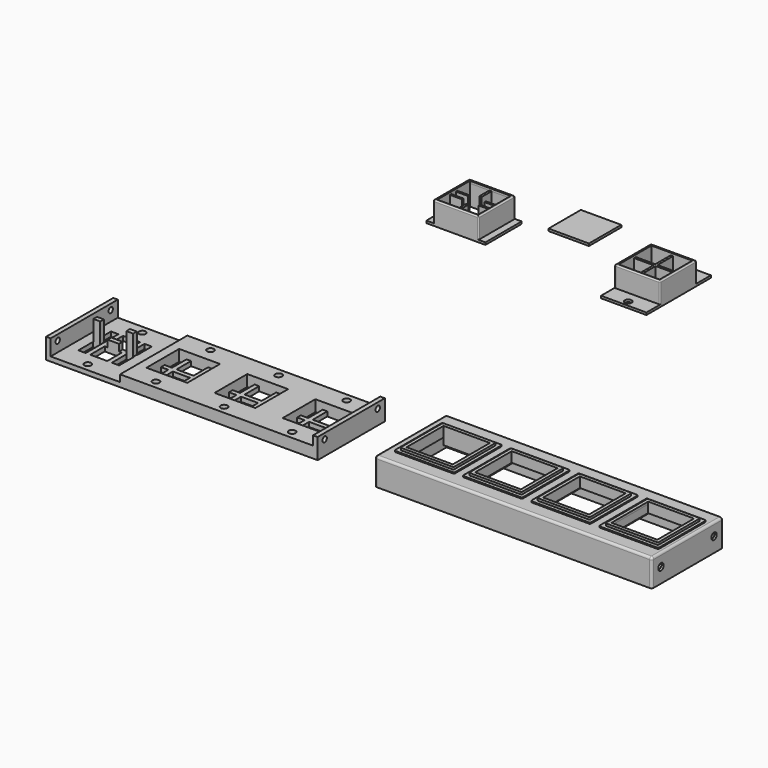
from build123d import *

# Parameters (mm, degrees)
F0_W          = 20
F0_H          = 20
F1_DEPTH      = 10
F2_T          = -1
F4_DEPTH      = 9
F5_W          = 20
F5_H          = 8
F5_R          = 1.5
F6_DEPTH      = 1
F7_W          = 20
F7_H          = 20
F8_DEPTH      = 10
F9_W          = 3
F9_H          = 20
F9_W_2        = 20
F10_DEPTH     = 0.95
F11_T         = 1
F11_T3_DEPTH  = 22
F12_W         = 8.5
F12_H         = 0.8
F13_DEPTH     = 9
F15_DEPTH     = 9
F16_W         = 117
F16_H         = 37
F16_R         = 1.5
F17_DEPTH     = 1
F18_W         = 122
F18_H         = 39.2
F18_W_2       = 20.4
F18_H_2       = 20.4
F18_W_3       = 20.2
F18_H_3       = 20.2
F19_DEPTH     = 11
F20_W         = 120
F20_H         = 37.2
F21_DEPTH     = 8
F22_W         = 4
F22_H         = 18
F23_DEPTH     = 3
F25_W         = 3
F25_H         = 2
F26_DEPTH     = 9
F27_W         = 5
F27_H         = 2
F28_DEPTH     = 3
F29_R         = 1
F30_R         = 0.5
F30_2_R       = 0.5
F24_R         = 1.5
F31_DEPTH     = 3
F32_DEPTH     = 2
F33_W         = 2
F33_H         = 37
F34_DEPTH     = 7
F35_W         = 20.4
F35_H         = 8.4
F36_DEPTH     = 3
F37_R         = 1.5
F38_DEPTH     = 3
F40_R         = 1.5
F41_DEPTH     = 2
F42_W         = 3
F42_H         = 37.2
F43_DEPTH     = 1
F44_DEPTH     = 1
F45_W         = 2
F45_H         = 37
F46_DEPTH     = 4
F39_R         = 1.2
F47_DEPTH     = 269.2358512024
F48_DEPTH     = 3
F49_DEPTH     = 5
F32_FACE2_W   = 119
F32_FACE2_H   = 37
F32_FACE2_R   = 1.5
F32_FACE2_W_2 = 3.25
F32_FACE2_H_2 = 8
F32_FACE2_W_3 = 7.5
F50_DEPTH     = 1
F51_DEPTH     = 1
F52_DEPTH     = 2
F53_DEPTH     = 0.05
F54_W         = 20.4
F54_H         = 3
F54_W_2       = 20.2
F54_H_2       = 3.1
F55_DEPTH     = 0.5
F56_W         = 20.4
F56_H         = 1.5
F56_W_2       = 20.2
F57_DEPTH     = 1
F58_R         = 0.5
F59_W         = 18
F59_H         = 17.9999990673
F60_DEPTH     = 1
F61_W         = 17.8
F61_H         = 17.8
F62_DEPTH     = 1
F63_W         = 18
F63_H         = 18
F64_DEPTH     = 1


# Not quite as in the source:
# - a shell that OpenCascade refuses in one call is made with other operations: the cavity is built on its own and cut out


with BuildPart() as f1:
    # F0 (on Top) → F1 (new body)
    with BuildSketch(Plane.XY):
        Rectangle(F0_W, F0_H)
    extrude(amount=F1_DEPTH)

    # F2
    f2_openings = [f1.faces().sort_by_distance(p)[0] for p in [
        (0, 0, 0),
    ]]
    offset(amount=F2_T, openings=f2_openings)

    # F3 (on Top) → F4 (join)
    with BuildSketch(Plane.XY):
        Polygon((-0.5, -9), (0.5, -9), (0.5, -0.5), (9, -0.5), (9, 0.5), (0.5, 0.5), (0.5, 9), (-0.5, 9), (-0.5, 0.5), (-9, 0.5), (-9, -0.5), (-0.5, -0.5), align=None)
    extrude(amount=F4_DEPTH)

    # F5 (on Top) → F6 (join)
    with BuildSketch(Plane.XY):
        with Locations((0, -13.5)):
            Rectangle(F5_W, F5_H)
        with Locations((0, -15)):
            Circle(F5_R, mode=Mode.SUBTRACT)
        with Locations((0, 14)):
            Rectangle(F5_W, F5_H)
        with Locations((0, 15)):
            Circle(F5_R, mode=Mode.SUBTRACT)
    extrude(amount=F6_DEPTH)

    # F30
    f30_edges = [f1.edges().sort_by_distance(p)[0] for p in [
        (-10, -10, 5.5),
        (0, -10, 10),
        (10, -10, 5.5),
        (-10, 0, 10),
        (-10, 10, 5.5),
        (0, 10, 10),
        (10, 10, 5.5),
        (10, 0, 10),
    ]]
    fillet(f30_edges, radius=F30_R)

    # F63 (on face) → F64 (cut)
    with BuildSketch(Plane.XY.offset(10)):
        Rectangle(F63_W, F63_H)
    extrude(amount=-F64_DEPTH, mode=Mode.SUBTRACT)


with BuildPart() as f8:
    # F7 (on Top) → F8 (new body)
    with BuildSketch(Plane.XY):
        with Locations((-78.8846665621, -1.3073290847)):
            Rectangle(F7_W, F7_H)
    extrude(amount=F8_DEPTH)

    # F9 (on face) → F10 (join)
    with BuildSketch(Plane(origin=(0, 0, 0), x_dir=(1, 0, 0), z_dir=(0, 0, -1))):
        with Locations((-90.3846665621, 1.3073290847)):
            Rectangle(F9_W, F9_H)
        with Locations((-78.8846665621, 1.3073290847)):
            Rectangle(F9_W_2, F9_H)
        with Locations((-67.3846665621, 1.3073290847)):
            Rectangle(F9_W, F9_H)
    extrude(amount=-F10_DEPTH)

    # F11: shell of thickness 1, made by hand


with BuildPart() as f11_core1:
    # F11_t2: copy of F8
    add(f8.part)

    # the walls: a layer under each face that stays
    f11_faces = [f11_core1.faces().sort_by_distance(p)[0] for p in [
        (-78.8846665621, 8.6926709153, 5),
        (-91.8846665621, -1.3073290847, 0.475),
        (-78.8846665621, -11.3073290847, 5),
        (-90.3846665621, -1.3073290847, 0.95),
        (-88.8846665621, -1.3073290847, 5.475),
        (-78.8846665621, -1.3073290847, 10),
        (-68.8846665621, -1.3073290847, 5.475),
        (-67.3846665621, -1.3073290847, 0.95),
        (-65.8846665621, -1.3073290847, 0.475),
    ]]
    thicken(f11_faces, amount=-F11_T, mode=Mode.SUBTRACT)

    # F11_s4 → F11_t3 (cut)
    with BuildSketch(Plane.XZ.offset(-9.6926709153)):
        Polygon((-88.8946665621, 0.96), (-88.8846665621, -0.05), (-87.8846665621, -0.05), (-87.8846665621, 0.95), align=None)
        Polygon((-68.8746665621, 0.96), (-69.8846665621, 0.95), (-69.8846665621, -0.05), (-68.8846665621, -0.05), align=None)
    extrude(amount=F11_T3_DEPTH, mode=Mode.SUBTRACT)


with BuildPart() as f8_1:
    add(f8.part)

    # what is left inside the walls is the cavity
    f11_cavity = [f11_core1.part.solids().sort_by_distance(p)[0] for p in [
        (-78.884667, -4.307329, 0.01),
    ]]
    add(f11_cavity, mode=Mode.SUBTRACT)

    # F12 (on Top) → F13 (join)
    with BuildSketch(Plane.XY):
        Polygon((-78.3846665621, 7.6926709153), (-79.3846665621, 7.6926709153), (-79.3846665621, 0.6926709153), (-79.3846665621, -0.1073290847), (-79.3846665621, -2.5073290847), (-79.3846665621, -3.3073290847), (-79.3846665621, -10.3073290847), (-78.3846665621, -10.3073290847), (-78.3846665621, -3.3073290847), (-78.3846665621, -2.5073290847), (-78.3846665621, -0.1073290847), (-78.3846665621, 0.6926709153), align=None)
        with Locations((-83.6346665621, -2.9073290847)):
            Rectangle(F12_W, F12_H)
        with Locations((-83.6346665621, 0.2926709153)):
            Rectangle(F12_W, F12_H)
        with Locations((-74.1346665621, 0.2926709153)):
            Rectangle(F12_W, F12_H)
        with Locations((-74.1346665621, -2.9073290847)):
            Rectangle(F12_W, F12_H)
    extrude(amount=F13_DEPTH)

    # F14 (on face) → F15 (cut)
    with BuildSketch(Plane(origin=(0, 0, 0), x_dir=(1, 0, 0), z_dir=(0, 0, -1))):
        Polygon((-79.3846665621, -2.2926709153), (-78.3846665621, -2.2926709153), (-78.3846665621, -0.6926709153), (-75.2846665621, -0.6926709153), (-75.2846665621, 0.1073290847), (-78.3846665621, 0.1073290847), (-78.3846665621, 2.5073290847), (-75.2846665621, 2.5073290847), (-75.2846665621, 3.3073290847), (-78.3846665621, 3.3073290847), (-78.3846665621, 4.9073290847), (-79.3846665621, 4.9073290847), (-79.3846665621, 3.3073290847), (-82.4846665621, 3.3073290847), (-82.4846665621, 2.5073290847), (-79.3846665621, 2.5073290847), (-79.3846665621, 0.1073290847), (-82.4846665621, 0.1073290847), (-82.4846665621, -0.6926709153), (-79.3846665621, -0.6926709153), align=None)
    extrude(amount=-F15_DEPTH, mode=Mode.SUBTRACT)

    # F30#2
    f30_2_edges = [f8_1.edges().sort_by_distance(p)[0] for p in [
        (-68.884667, -11.307329, 5.475),
        (-78.884667, -11.307329, 10),
        (-68.884667, -1.307329, 10),
        (-68.884667, 8.692671, 5.475),
        (-78.884667, 8.692671, 10),
        (-88.884667, 8.692671, 5.475),
        (-88.884667, -1.307329, 10),
        (-88.884667, -11.307329, 5.475),
    ]]
    fillet(f30_2_edges, radius=F30_2_R)

    # F53 (add): faces of the model
    f53_faces = [f8_1.faces().sort_by_distance(p)[0] for p in [
        (-90.3817894545, -1.3073290847, 0.95),
        (-67.3875436696, -1.3073290847, 0.95),
    ]]
    extrude(f53_faces, amount=F53_DEPTH)

    # F59 (on face) → F60 (cut)
    with BuildSketch(Plane.XY.offset(10)):
        with Locations((-78.8846665621, -1.3073295511)):
            Rectangle(F59_W, F59_H)
    extrude(amount=-F60_DEPTH, mode=Mode.SUBTRACT)


with BuildPart() as f17:
    # F16 (on Top) → F17 (new body)
    with BuildSketch(Plane.XY):
        with Locations((-71.0754835367, -152.5580135584)):
            Rectangle(F16_W, F16_H)
        with Locations((-115.9754835367, -167.5580135584)):
            Circle(F16_R, mode=Mode.SUBTRACT)
        with Locations((-85.9754835367, -167.5580135584)):
            Circle(F16_R, mode=Mode.SUBTRACT)
        Polygon((-124.9754835367, -151.5580135584), (-124.9754835367, -143.5580135584), (-121.7254835367, -143.5580135584), (-119.7254835367, -143.5580135584), (-112.2254835367, -143.5580135584), (-110.2254835367, -143.5580135584), (-106.9754835367, -143.5580135584), (-106.9754835367, -151.5580135584), (-106.9754835367, -153.5580135584), (-106.9754835367, -161.5580135584), (-110.2254835367, -161.5580135584), (-112.2254835367, -161.5580135584), (-119.7254835367, -161.5580135584), (-121.7254835367, -161.5580135584), (-124.9754835367, -161.5580135584), (-124.9754835367, -153.5580135584), align=None, mode=Mode.SUBTRACT)
        Polygon((-94.9754835367, -151.5580135584), (-94.9754835367, -143.5580135584), (-91.7254835367, -143.5580135584), (-89.7254835367, -143.5580135584), (-82.2254835367, -143.5580135584), (-80.2254835367, -143.5580135584), (-76.9754835367, -143.5580135584), (-76.9754835367, -151.5580135584), (-76.9754835367, -153.5580135584), (-76.9754835367, -161.5580135584), (-80.2254835367, -161.5580135584), (-82.2254835367, -161.5580135584), (-89.7254835367, -161.5580135584), (-91.7254835367, -161.5580135584), (-94.9754835367, -161.5580135584), (-94.9754835367, -153.5580135584), align=None, mode=Mode.SUBTRACT)
        with Locations((-55.9754835367, -167.5580135584)):
            Circle(F16_R, mode=Mode.SUBTRACT)
        with Locations((-25.9754835367, -167.5580135584)):
            Circle(F16_R, mode=Mode.SUBTRACT)
        Polygon((-64.9754835367, -151.5580135584), (-64.9754835367, -143.5580135584), (-61.7254835367, -143.5580135584), (-59.7254835367, -143.5580135584), (-52.2254835367, -143.5580135584), (-50.2254835367, -143.5580135584), (-46.9754835367, -143.5580135584), (-46.9754835367, -151.5580135584), (-46.9754835367, -153.5580135584), (-46.9754835367, -161.5580135584), (-47.9754835367, -161.5580135584), (-50.2254835367, -161.5580135584), (-52.2254835367, -161.5580135584), (-59.7254835367, -161.5580135584), (-61.7254835367, -161.5580135584), (-64.9754835367, -161.5580135584), (-64.9754835367, -153.5580135584), align=None, mode=Mode.SUBTRACT)
        Polygon((-34.9754835367, -151.5580135584), (-34.9754835367, -143.5580135584), (-31.7254835367, -143.5580135584), (-29.7254835367, -143.5580135584), (-22.2254835367, -143.5580135584), (-20.2254835367, -143.5580135584), (-16.9754835367, -143.5580135584), (-16.9754835367, -151.5580135584), (-16.9754835367, -153.5580135584), (-16.9754835367, -161.5580135584), (-17.9754835367, -161.5580135584), (-20.2254835367, -161.5580135584), (-22.2254835367, -161.5580135584), (-29.7254835367, -161.5580135584), (-31.7254835367, -161.5580135584), (-34.9754835367, -161.5580135584), (-34.9754835367, -153.5580135584), align=None, mode=Mode.SUBTRACT)
        with Locations((-115.9754835367, -137.5580135584)):
            Circle(F16_R, mode=Mode.SUBTRACT)
        with Locations((-85.9754835367, -137.5580135584)):
            Circle(F16_R, mode=Mode.SUBTRACT)
        with Locations((-55.9754835367, -137.5580135584)):
            Circle(F16_R, mode=Mode.SUBTRACT)
        with Locations((-25.9754835367, -137.5580135584)):
            Circle(F16_R, mode=Mode.SUBTRACT)
        Polygon((-119.7254835367, -143.5580135584), (-121.7254835367, -143.5580135584), (-121.7254835367, -151.5580135584), (-124.9754835367, -151.5580135584), (-124.9754835367, -153.5580135584), (-121.7254835367, -153.5580135584), (-121.7254835367, -161.5580135584), (-119.7254835367, -161.5580135584), (-119.7254835367, -153.5580135584), (-112.2254835367, -153.5580135584), (-112.2254835367, -161.5580135584), (-110.2254835367, -161.5580135584), (-110.2254835367, -153.5580135584), (-106.9754835367, -153.5580135584), (-106.9754835367, -151.5580135584), (-110.2254835367, -151.5580135584), (-110.2254835367, -143.5580135584), (-112.2254835367, -143.5580135584), (-112.2254835367, -151.5580135584), (-119.7254835367, -151.5580135584), align=None)
        Polygon((-89.7254835367, -143.5580135584), (-91.7254835367, -143.5580135584), (-91.7254835367, -151.5580135584), (-94.9754835367, -151.5580135584), (-94.9754835367, -153.5580135584), (-91.7254835367, -153.5580135584), (-91.7254835367, -161.5580135584), (-89.7254835367, -161.5580135584), (-89.7254835367, -153.5580135584), (-82.2254835367, -153.5580135584), (-82.2254835367, -161.5580135584), (-80.2254835367, -161.5580135584), (-80.2254835367, -153.5580135584), (-76.9754835367, -153.5580135584), (-76.9754835367, -151.5580135584), (-80.2254835367, -151.5580135584), (-80.2254835367, -143.5580135584), (-82.2254835367, -143.5580135584), (-82.2254835367, -151.5580135584), (-89.7254835367, -151.5580135584), align=None)
        Polygon((-59.7254835367, -143.5580135584), (-61.7254835367, -143.5580135584), (-61.7254835367, -151.5580135584), (-64.9754835367, -151.5580135584), (-64.9754835367, -153.5580135584), (-61.7254835367, -153.5580135584), (-61.7254835367, -161.5580135584), (-59.7254835367, -161.5580135584), (-59.7254835367, -153.5580135584), (-52.2254835367, -153.5580135584), (-52.2254835367, -161.5580135584), (-50.2254835367, -161.5580135584), (-50.2254835367, -153.5580135584), (-46.9754835367, -153.5580135584), (-46.9754835367, -151.5580135584), (-50.2254835367, -151.5580135584), (-50.2254835367, -143.5580135584), (-52.2254835367, -143.5580135584), (-52.2254835367, -151.5580135584), (-59.7254835367, -151.5580135584), align=None)
        Polygon((-29.7254835367, -143.5580135584), (-31.7254835367, -143.5580135584), (-31.7254835367, -151.5580135584), (-34.9754835367, -151.5580135584), (-34.9754835367, -153.5580135584), (-31.7254835367, -153.5580135584), (-31.7254835367, -161.5580135584), (-29.7254835367, -161.5580135584), (-29.7254835367, -153.5580135584), (-22.2254835367, -153.5580135584), (-22.2254835367, -161.5580135584), (-20.2254835367, -161.5580135584), (-20.2254835367, -153.5580135584), (-16.9754835367, -153.5580135584), (-16.9754835367, -151.5580135584), (-20.2254835367, -151.5580135584), (-20.2254835367, -143.5580135584), (-22.2254835367, -143.5580135584), (-22.2254835367, -151.5580135584), (-29.7254835367, -151.5580135584), align=None)
    extrude(amount=F17_DEPTH)

    # F22 (on face) → F23 (join)
    with BuildSketch(Plane.XY.offset(1)):
        with Locations((-96.9754835367, -152.5580135584)):
            Rectangle(F22_W, F22_H)
        with Locations((-74.9754835367, -152.5580135584)):
            Rectangle(F22_W, F22_H)
        with Locations((-66.9754835367, -152.5580135584)):
            Rectangle(F22_W, F22_H)
        with Locations((-44.9754835367, -152.5580135584)):
            Rectangle(F22_W, F22_H)
        with Locations((-36.9754835367, -152.5580135584)):
            Rectangle(F22_W, F22_H)
        with Locations((-14.9754835367, -152.5580135584)):
            Rectangle(F22_W, F22_H)
    extrude(amount=F23_DEPTH)

    # F25 (on face) → F26 (join)
    with BuildSketch(Plane.XY.offset(1)):
        with Locations((-123.2254835367, -152.5580135584)):
            Rectangle(F25_W, F25_H)
        with Locations((-108.7254835367, -152.5580135584)):
            Rectangle(F25_W, F25_H)
    extrude(amount=F26_DEPTH)

    # F27 (on face) → F28 (join)
    with BuildSketch(Plane.XY.offset(1)):
        with Locations((-115.9754835367, -152.5580135584)):
            Rectangle(F27_W, F27_H)
    extrude(amount=F28_DEPTH)

    # F24 (on face) → F31 (join)
    with BuildSketch(Plane.XY.offset(1)):
        Polygon((-98.9754835367, -134.0580135584), (-98.9754835367, -143.5580135584), (-94.9754835367, -143.5580135584), (-91.7254835367, -143.5580135584), (-89.7254835367, -143.5580135584), (-82.2254835367, -143.5580135584), (-80.2254835367, -143.5580135584), (-76.9754835367, -143.5580135584), (-72.9754835367, -143.5580135584), (-72.9754835367, -134.0580135584), align=None)
        with Locations((-85.9754835367, -137.5580135584)):
            Circle(F24_R, mode=Mode.SUBTRACT)
        Polygon((-94.9754835367, -161.5580135584), (-98.9754835367, -161.5580135584), (-98.9754835367, -171.0580135584), (-72.9754835367, -171.0580135584), (-72.9754835367, -161.5580135584), (-76.9754835367, -161.5580135584), (-80.2254835367, -161.5580135584), (-82.2254835367, -161.5580135584), (-89.7254835367, -161.5580135584), (-91.7254835367, -161.5580135584), align=None)
        with Locations((-85.9754835367, -167.5580135584)):
            Circle(F24_R, mode=Mode.SUBTRACT)
        Polygon((-68.9754835367, -161.5580135584), (-68.9754835367, -171.0580135584), (-42.9754835367, -171.0580135584), (-42.9754835367, -161.5580135584), (-46.9754835367, -161.5580135584), (-50.2254835367, -161.5580135584), (-52.2254835367, -161.5580135584), (-59.7254835367, -161.5580135584), (-61.7254835367, -161.5580135584), (-64.9754835367, -161.5580135584), align=None)
        with Locations((-55.9754835367, -167.5580135584)):
            Circle(F24_R, mode=Mode.SUBTRACT)
        Polygon((-42.9754835367, -134.0580135584), (-68.9754835367, -134.0580135584), (-68.9754835367, -143.5580135584), (-64.9754835367, -143.5580135584), (-61.7254835367, -143.5580135584), (-59.7254835367, -143.5580135584), (-52.2254835367, -143.5580135584), (-50.2254835367, -143.5580135584), (-46.9754835367, -143.5580135584), (-42.9754835367, -143.5580135584), align=None)
        with Locations((-55.9754835367, -137.5580135584)):
            Circle(F24_R, mode=Mode.SUBTRACT)
        Polygon((-12.9754835367, -134.0580135584), (-38.9754835367, -134.0580135584), (-38.9754835367, -143.5580135584), (-34.9754835367, -143.5580135584), (-31.7254835367, -143.5580135584), (-29.7254835367, -143.5580135584), (-22.2254835367, -143.5580135584), (-20.2254835367, -143.5580135584), (-16.9754835367, -143.5580135584), (-12.9754835367, -143.5580135584), align=None)
        with Locations((-25.9754835367, -137.5580135584)):
            Circle(F24_R, mode=Mode.SUBTRACT)
        Polygon((-38.9754835367, -161.5580135584), (-38.9754835367, -171.0580135584), (-12.9754835367, -171.0580135584), (-12.9754835367, -161.5580135584), (-16.9754835367, -161.5580135584), (-20.2254835367, -161.5580135584), (-22.2254835367, -161.5580135584), (-29.7254835367, -161.5580135584), (-31.7254835367, -161.5580135584), (-34.9754835367, -161.5580135584), align=None)
        with Locations((-25.9754835367, -167.5580135584)):
            Circle(F24_R, mode=Mode.SUBTRACT)
    extrude(amount=F31_DEPTH)

    # F32 (add): a face of the model
    f32_faces = [f17.faces().sort_by_distance(p)[0] for p in [
        (-129.5754835367, -152.5580135584, 0.5),
    ]]
    extrude(f32_faces, amount=F32_DEPTH)

    # F33 (on face) → F34 (join)
    with BuildSketch(Plane.XY.offset(1)):
        with Locations((-130.5754835367, -152.5580135584)):
            Rectangle(F33_W, F33_H)
    extrude(amount=F34_DEPTH)

    # F44 (add): a face of the model
    f44_faces = [f17.faces().sort_by_distance(p)[0] for p in [
        (-12.9754835367, -152.5580135584, 2.5),
    ]]
    extrude(f44_faces, amount=F44_DEPTH)

    # F45 (on face) → F46 (join)
    with BuildSketch(Plane.XY.offset(4)):
        with Locations((-12.9754835367, -152.5580135584)):
            Rectangle(F45_W, F45_H)
    extrude(amount=F46_DEPTH)

    # F39 (on face) → F47 (cut, through all)
    with BuildSketch(Plane(origin=(-131.5754835367, 0, 0), x_dir=(0, -1, 0), z_dir=(-1, 0, 0))):
        with Locations((137.9580135584, 5.5)):
            Circle(F39_R)
        with Locations((167.1580135584, 5.5)):
            Circle(F39_R)
    extrude(amount=-F47_DEPTH, mode=Mode.SUBTRACT)

    # F49 (add): faces of the model
    f49_faces = [f17.faces().sort_by_distance(p)[0] for p in [
        (-72.9754835367, -152.5580135584, 2.5),
        (-42.9754835367, -152.5580135584, 2.5),
    ]]
    extrude(f49_faces, amount=F49_DEPTH)

    # F16 (on Top) + F32_face2 (on face) → F50 (join)
    with BuildSketch(Plane.XY):
        with Locations((-71.0754835367, -152.5580135584)):
            Rectangle(F16_W, F16_H)
        with Locations((-115.9754835367, -167.5580135584)):
            Circle(F16_R, mode=Mode.SUBTRACT)
        with Locations((-85.9754835367, -167.5580135584)):
            Circle(F16_R, mode=Mode.SUBTRACT)
        Polygon((-124.9754835367, -151.5580135584), (-124.9754835367, -143.5580135584), (-121.7254835367, -143.5580135584), (-119.7254835367, -143.5580135584), (-112.2254835367, -143.5580135584), (-110.2254835367, -143.5580135584), (-106.9754835367, -143.5580135584), (-106.9754835367, -151.5580135584), (-106.9754835367, -153.5580135584), (-106.9754835367, -161.5580135584), (-110.2254835367, -161.5580135584), (-112.2254835367, -161.5580135584), (-119.7254835367, -161.5580135584), (-121.7254835367, -161.5580135584), (-124.9754835367, -161.5580135584), (-124.9754835367, -153.5580135584), align=None, mode=Mode.SUBTRACT)
        Polygon((-94.9754835367, -151.5580135584), (-94.9754835367, -143.5580135584), (-91.7254835367, -143.5580135584), (-89.7254835367, -143.5580135584), (-82.2254835367, -143.5580135584), (-80.2254835367, -143.5580135584), (-76.9754835367, -143.5580135584), (-76.9754835367, -151.5580135584), (-76.9754835367, -153.5580135584), (-76.9754835367, -161.5580135584), (-80.2254835367, -161.5580135584), (-82.2254835367, -161.5580135584), (-89.7254835367, -161.5580135584), (-91.7254835367, -161.5580135584), (-94.9754835367, -161.5580135584), (-94.9754835367, -153.5580135584), align=None, mode=Mode.SUBTRACT)
        with Locations((-55.9754835367, -167.5580135584)):
            Circle(F16_R, mode=Mode.SUBTRACT)
        with Locations((-25.9754835367, -167.5580135584)):
            Circle(F16_R, mode=Mode.SUBTRACT)
        Polygon((-64.9754835367, -151.5580135584), (-64.9754835367, -143.5580135584), (-61.7254835367, -143.5580135584), (-59.7254835367, -143.5580135584), (-52.2254835367, -143.5580135584), (-50.2254835367, -143.5580135584), (-46.9754835367, -143.5580135584), (-46.9754835367, -151.5580135584), (-46.9754835367, -153.5580135584), (-46.9754835367, -161.5580135584), (-47.9754835367, -161.5580135584), (-50.2254835367, -161.5580135584), (-52.2254835367, -161.5580135584), (-59.7254835367, -161.5580135584), (-61.7254835367, -161.5580135584), (-64.9754835367, -161.5580135584), (-64.9754835367, -153.5580135584), align=None, mode=Mode.SUBTRACT)
        Polygon((-34.9754835367, -151.5580135584), (-34.9754835367, -143.5580135584), (-31.7254835367, -143.5580135584), (-29.7254835367, -143.5580135584), (-22.2254835367, -143.5580135584), (-20.2254835367, -143.5580135584), (-16.9754835367, -143.5580135584), (-16.9754835367, -151.5580135584), (-16.9754835367, -153.5580135584), (-16.9754835367, -161.5580135584), (-17.9754835367, -161.5580135584), (-20.2254835367, -161.5580135584), (-22.2254835367, -161.5580135584), (-29.7254835367, -161.5580135584), (-31.7254835367, -161.5580135584), (-34.9754835367, -161.5580135584), (-34.9754835367, -153.5580135584), align=None, mode=Mode.SUBTRACT)
        with Locations((-115.9754835367, -137.5580135584)):
            Circle(F16_R, mode=Mode.SUBTRACT)
        with Locations((-85.9754835367, -137.5580135584)):
            Circle(F16_R, mode=Mode.SUBTRACT)
        with Locations((-55.9754835367, -137.5580135584)):
            Circle(F16_R, mode=Mode.SUBTRACT)
        with Locations((-25.9754835367, -137.5580135584)):
            Circle(F16_R, mode=Mode.SUBTRACT)
    with BuildSketch(Plane(origin=(-72.3791549796, -152.5580135584, 0), x_dir=(1, 0, 0), z_dir=(0, 0, -1))):
        with Locations((0.3036714428, 0)):
            Rectangle(F32_FACE2_W, F32_FACE2_H)
        with Locations((-43.5963285572, 15)):
            Circle(F32_FACE2_R, mode=Mode.SUBTRACT)
        with Locations((-13.5963285572, 15)):
            Circle(F32_FACE2_R, mode=Mode.SUBTRACT)
        with Locations((-36.2213285572, 5)):
            Rectangle(F32_FACE2_W_2, F32_FACE2_H_2, mode=Mode.SUBTRACT)
        with Locations((-43.5963285572, 5)):
            Rectangle(F32_FACE2_W_3, F32_FACE2_H_2, mode=Mode.SUBTRACT)
        with Locations((-50.9713285572, 5)):
            Rectangle(F32_FACE2_W_2, F32_FACE2_H_2, mode=Mode.SUBTRACT)
        with Locations((-50.9713285572, -5)):
            Rectangle(F32_FACE2_W_2, F32_FACE2_H_2, mode=Mode.SUBTRACT)
        with Locations((-43.5963285572, -5)):
            Rectangle(F32_FACE2_W_3, F32_FACE2_H_2, mode=Mode.SUBTRACT)
        with Locations((-36.2213285572, -5)):
            Rectangle(F32_FACE2_W_2, F32_FACE2_H_2, mode=Mode.SUBTRACT)
        with Locations((-6.2213285572, 5)):
            Rectangle(F32_FACE2_W_2, F32_FACE2_H_2, mode=Mode.SUBTRACT)
        with Locations((-13.5963285572, 5)):
            Rectangle(F32_FACE2_W_3, F32_FACE2_H_2, mode=Mode.SUBTRACT)
        with Locations((-20.9713285572, 5)):
            Rectangle(F32_FACE2_W_2, F32_FACE2_H_2, mode=Mode.SUBTRACT)
        with Locations((-20.9713285572, -5)):
            Rectangle(F32_FACE2_W_2, F32_FACE2_H_2, mode=Mode.SUBTRACT)
        with Locations((-13.5963285572, -5)):
            Rectangle(F32_FACE2_W_3, F32_FACE2_H_2, mode=Mode.SUBTRACT)
        with Locations((-6.2213285572, -5)):
            Rectangle(F32_FACE2_W_2, F32_FACE2_H_2, mode=Mode.SUBTRACT)
        with Locations((16.4036714428, 15)):
            Circle(F32_FACE2_R, mode=Mode.SUBTRACT)
        with Locations((46.4036714428, 15)):
            Circle(F32_FACE2_R, mode=Mode.SUBTRACT)
        with Locations((23.7786714428, 5)):
            Rectangle(F32_FACE2_W_2, F32_FACE2_H_2, mode=Mode.SUBTRACT)
        with Locations((16.4036714428, 5)):
            Rectangle(F32_FACE2_W_3, F32_FACE2_H_2, mode=Mode.SUBTRACT)
        with Locations((9.0286714428, 5)):
            Rectangle(F32_FACE2_W_2, F32_FACE2_H_2, mode=Mode.SUBTRACT)
        with Locations((9.0286714428, -5)):
            Rectangle(F32_FACE2_W_2, F32_FACE2_H_2, mode=Mode.SUBTRACT)
        with Locations((16.4036714428, -5)):
            Rectangle(F32_FACE2_W_3, F32_FACE2_H_2, mode=Mode.SUBTRACT)
        with Locations((23.7786714428, -5)):
            Rectangle(F32_FACE2_W_2, F32_FACE2_H_2, mode=Mode.SUBTRACT)
        with Locations((53.7786714428, 5)):
            Rectangle(F32_FACE2_W_2, F32_FACE2_H_2, mode=Mode.SUBTRACT)
        with Locations((46.4036714428, 5)):
            Rectangle(F32_FACE2_W_3, F32_FACE2_H_2, mode=Mode.SUBTRACT)
        with Locations((39.0286714428, 5)):
            Rectangle(F32_FACE2_W_2, F32_FACE2_H_2, mode=Mode.SUBTRACT)
        with Locations((39.0286714428, -5)):
            Rectangle(F32_FACE2_W_2, F32_FACE2_H_2, mode=Mode.SUBTRACT)
        with Locations((46.4036714428, -5)):
            Rectangle(F32_FACE2_W_3, F32_FACE2_H_2, mode=Mode.SUBTRACT)
        with Locations((53.7786714428, -5)):
            Rectangle(F32_FACE2_W_2, F32_FACE2_H_2, mode=Mode.SUBTRACT)
        with Locations((-43.5963285572, -15)):
            Circle(F32_FACE2_R, mode=Mode.SUBTRACT)
        with Locations((-13.5963285572, -15)):
            Circle(F32_FACE2_R, mode=Mode.SUBTRACT)
        with Locations((16.4036714428, -15)):
            Circle(F32_FACE2_R, mode=Mode.SUBTRACT)
        with Locations((46.4036714428, -15)):
            Circle(F32_FACE2_R, mode=Mode.SUBTRACT)
    extrude(amount=-F50_DEPTH, dir=(0, 0, 1))

    # F52 (add): a face of the model
    f52_faces = [f17.faces().sort_by_distance(p)[0] for p in [
        (-12.2754835367, -152.5580135584, 1),
    ]]
    extrude(f52_faces, amount=F52_DEPTH)


with BuildPart() as f19:
    # F18 (on Top) → F19 (new body)
    with BuildSketch(Plane.XY):
        with Locations((76.6593676656, -154.4580135584)):
            Rectangle(F18_W, F18_H)
        with Locations((32.2593676656, -154.4580135584)):
            Rectangle(F18_W_2, F18_H_2, mode=Mode.SUBTRACT)
        with Locations((62.2593676656, -154.4580135584)):
            Rectangle(F18_W_3, F18_H_3, mode=Mode.SUBTRACT)
        with Locations((92.2593676656, -154.4580135584)):
            Rectangle(F18_W_3, F18_H_3, mode=Mode.SUBTRACT)
        with Locations((122.2593676656, -154.4580135584)):
            Rectangle(F18_W_3, F18_H_3, mode=Mode.SUBTRACT)
    extrude(amount=F19_DEPTH)

    # F20 (on face) → F21 (cut)
    with BuildSketch(Plane(origin=(0, 0, 0), x_dir=(1, 0, 0), z_dir=(0, 0, -1))):
        with Locations((76.6593676656, 154.4580135584)):
            Rectangle(F20_W, F20_H)
    extrude(amount=-F21_DEPTH, mode=Mode.SUBTRACT)

    # F29
    f29_edges = [f19.edges().sort_by_distance(p)[0] for p in [
        (15.659368, -134.858014, 5.5),
        (15.659368, -174.058014, 5.5),
        (137.659368, -174.058014, 5.5),
        (137.659368, -134.858014, 5.5),
        (76.659368, -174.058014, 11),
        (15.659368, -154.458014, 11),
        (76.659368, -134.858014, 11),
        (137.659368, -154.458014, 11),
    ]]
    fillet(f29_edges, radius=F29_R)

    # F35 (on face) → F36 (join)
    with BuildSketch(Plane(origin=(0, 0, 8), x_dir=(1, 0, 0), z_dir=(0, 0, -1))):
        with Locations((32.2593676656, 168.8580135584)):
            Rectangle(F35_W, F35_H)
        with Locations((32.2593676656, 140.0580135584)):
            Rectangle(F35_W, F35_H)
    extrude(amount=F36_DEPTH)

    # F37 (on face) → F38 (cut)
    with BuildSketch(Plane(origin=(15.6593676656, 0, 0), x_dir=(0, -1, 0), z_dir=(-1, 0, 0))):
        with Locations((139.8580135584, 5.5)):
            Circle(F37_R)
        with Locations((169.0580135584, 5.5)):
            Circle(F37_R)
    extrude(amount=-F38_DEPTH, mode=Mode.SUBTRACT)

    # F40 (on face) → F41 (cut)
    with BuildSketch(Plane.YZ.offset(137.6593676656)):
        with Locations((-169.0580135584, 5.5)):
            Circle(F40_R)
        with Locations((-139.8580135584, 5.5)):
            Circle(F40_R)
    extrude(amount=-F41_DEPTH, mode=Mode.SUBTRACT)

    # F42 (on face) → F43 (join)
    with BuildSketch(Plane(origin=(0, 0, 8), x_dir=(1, 0, 0), z_dir=(0, 0, -1))):
        with Locations((47.4593676656, 154.4580135584)):
            Rectangle(F42_W, F42_H)
        with Locations((77.3593676656, 154.4580135584)):
            Rectangle(F42_W, F42_H)
        with Locations((107.3593676656, 154.4580135584)):
            Rectangle(F42_W, F42_H)
    extrude(amount=F43_DEPTH)

    # F42 (on face) → F48 (join)
    with BuildSketch(Plane(origin=(0, 0, 8), x_dir=(1, 0, 0), z_dir=(0, 0, -1))):
        with Locations((47.4593676656, 154.4580135584)):
            Rectangle(F42_W, F42_H)
        with Locations((77.3593676656, 154.4580135584)):
            Rectangle(F42_W, F42_H)
        with Locations((107.3593676656, 154.4580135584)):
            Rectangle(F42_W, F42_H)
    extrude(amount=F48_DEPTH)

    # F51 (add): a face of the model
    f51_faces = [f19.faces().sort_by_distance(p)[0] for p in [
        (137.5312246206, -154.4580135584, 0),
    ]]
    extrude(f51_faces, amount=F51_DEPTH)

    # F54 (on face) → F55 (join)
    with BuildSketch(Plane.XY.offset(11)):
        with Locations((32.2593676656, -142.7580135584)):
            Rectangle(F54_W, F54_H)
        Polygon((22.0593676656, -164.6580135584), (22.0593676656, -144.2580135584), (22.0593676656, -141.2580135584), (19.0593676656, -141.2580135584), (19.0593676656, -167.6580135584), (22.0593676656, -167.6580135584), align=None)
        Polygon((42.4593676656, -141.2580135584), (42.4593676656, -144.2580135584), (42.4593676656, -164.6580135584), (42.4593676656, -167.6580135584), (45.4593676656, -167.6580135584), (45.4593676656, -141.2580135584), align=None)
        with Locations((32.2593676656, -166.1580135584)):
            Rectangle(F54_W, F54_H)
        with Locations((62.2593676656, -142.8080135584)):
            Rectangle(F54_W_2, F54_H_2)
        Polygon((52.1593676656, -164.5580135584), (52.1593676656, -144.3580135584), (52.1593676656, -141.2580135584), (49.1593676656, -141.2580135584), (49.1593676656, -167.6580135584), (52.1593676656, -167.6580135584), align=None)
        Polygon((72.3593676656, -141.2580135584), (72.3593676656, -144.3580135584), (72.3593676656, -164.5580135584), (72.3593676656, -167.6580135584), (75.3593676656, -167.6580135584), (75.3593676656, -141.2580135584), align=None)
        with Locations((62.2593676656, -166.1080135584)):
            Rectangle(F54_W_2, F54_H_2)
        with Locations((92.2593676656, -142.8080135584)):
            Rectangle(F54_W_2, F54_H_2)
        Polygon((82.1593676656, -164.5580135584), (82.1593676656, -144.3580135584), (82.1593676656, -141.2580135584), (79.1593676656, -141.2580135584), (79.1593676656, -167.6580135584), (82.1593676656, -167.6580135584), align=None)
        Polygon((102.3593676656, -141.2580135584), (102.3593676656, -144.3580135584), (102.3593676656, -164.5580135584), (102.3593676656, -167.6580135584), (105.3593676656, -167.6580135584), (105.3593676656, -141.2580135584), align=None)
        with Locations((92.2593676656, -166.1080135584)):
            Rectangle(F54_W_2, F54_H_2)
        with Locations((122.2593676656, -142.8080135584)):
            Rectangle(F54_W_2, F54_H_2)
        Polygon((112.1593676656, -164.5580135584), (112.1593676656, -144.3580135584), (112.1593676656, -141.2580135584), (109.1593676656, -141.2580135584), (109.1593676656, -167.6580135584), (112.1593676656, -167.6580135584), align=None)
        Polygon((132.3593676656, -141.2580135584), (132.3593676656, -144.3580135584), (132.3593676656, -164.5580135584), (132.3593676656, -167.6580135584), (135.3593676656, -167.6580135584), (135.3593676656, -141.2580135584), align=None)
        with Locations((122.2593676656, -166.1080135584)):
            Rectangle(F54_W_2, F54_H_2)
    extrude(amount=F55_DEPTH)

    # F56 (on face) → F57 (join)
    with BuildSketch(Plane.XY.offset(11.5)):
        with Locations((32.2593676656, -143.5080135584)):
            Rectangle(F56_W, F56_H)
        Polygon((22.0593676656, -164.6580135584), (22.0593676656, -144.2580135584), (22.0593676656, -142.7580135584), (20.5593676656, -142.7580135584), (20.5593676656, -166.1580135584), (22.0593676656, -166.1580135584), align=None)
        Polygon((42.4593676656, -142.7580135584), (42.4593676656, -144.2580135584), (42.4593676656, -164.6580135584), (42.4593676656, -166.1580135584), (43.9593676656, -166.1580135584), (43.9593676656, -142.7580135584), align=None)
        with Locations((32.2593676656, -165.4080135584)):
            Rectangle(F56_W, F56_H)
        Polygon((52.1593676656, -142.8580135584), (50.6593676656, -142.8580135584), (50.6593676656, -166.0580135584), (52.1593676656, -166.0580135584), (52.1593676656, -164.5580135584), (52.1593676656, -144.3580135584), align=None)
        with Locations((62.2593676656, -143.6080135584)):
            Rectangle(F56_W_2, F56_H)
        Polygon((73.8593676656, -142.8580135584), (72.3593676656, -142.8580135584), (72.3593676656, -144.3580135584), (72.3593676656, -164.5580135584), (72.3593676656, -166.0580135584), (73.8593676656, -166.0580135584), align=None)
        with Locations((62.2593676656, -165.3080135584)):
            Rectangle(F56_W_2, F56_H)
        Polygon((82.1593676656, -142.8580135584), (80.6593676656, -142.8580135584), (80.6593676656, -166.0580135584), (82.1593676656, -166.0580135584), (82.1593676656, -164.5580135584), (82.1593676656, -144.3580135584), align=None)
        with Locations((92.2593676656, -143.6080135584)):
            Rectangle(F56_W_2, F56_H)
        Polygon((103.8593676656, -142.8580135584), (102.3593676656, -142.8580135584), (102.3593676656, -144.3580135584), (102.3593676656, -164.5580135584), (102.3593676656, -166.0580135584), (103.8593676656, -166.0580135584), align=None)
        with Locations((92.2593676656, -165.3080135584)):
            Rectangle(F56_W_2, F56_H)
        Polygon((112.2593676656, -142.8580135584), (110.7593676656, -142.8580135584), (110.7593676656, -166.0580135584), (112.2593676656, -166.0580135584), (112.2593676656, -164.5580135584), (112.2593676656, -144.3580135584), align=None)
        with Locations((122.3593676656, -143.6080135584)):
            Rectangle(F56_W_2, F56_H)
        Polygon((133.9593676656, -142.8580135584), (132.4593676656, -142.8580135584), (132.4593676656, -144.3580135584), (132.4593676656, -164.5580135584), (132.4593676656, -166.0580135584), (133.9593676656, -166.0580135584), align=None)
        with Locations((122.3593676656, -165.3080135584)):
            Rectangle(F56_W_2, F56_H)
    extrude(amount=F57_DEPTH)

    # F58
    f58_edges = [f19.edges().sort_by_distance(p)[0] for p in [
        (19.059368, -141.258014, 11.25),
        (20.559368, -142.758014, 12),
        (19.059368, -167.658014, 11.25),
        (20.559368, -166.158014, 12),
        (43.959368, -166.158014, 12),
        (45.459368, -167.658014, 11.25),
        (43.959368, -142.758014, 12),
        (45.459368, -141.258014, 11.25),
        (49.159368, -141.258014, 11.25),
        (50.659368, -142.858014, 12),
        (50.659368, -166.058014, 12),
        (49.159368, -167.658014, 11.25),
        (73.859368, -166.058014, 12),
        (75.359368, -167.658014, 11.25),
        (73.859368, -142.858014, 12),
        (75.359368, -141.258014, 11.25),
        (79.159368, -141.258014, 11.25),
        (80.659368, -142.858014, 12),
        (79.159368, -167.658014, 11.25),
        (80.659368, -166.058014, 12),
        (103.859368, -166.058014, 12),
        (105.359368, -167.658014, 11.25),
        (103.859368, -142.858014, 12),
        (105.359368, -141.258014, 11.25),
        (109.159368, -141.258014, 11.25),
        (110.759368, -142.858014, 12),
        (109.159368, -167.658014, 11.25),
        (110.759368, -166.058014, 12),
        (133.959368, -166.058014, 12),
        (135.359368, -167.658014, 11.25),
        (133.959368, -142.858014, 12),
        (135.359368, -141.258014, 11.25),
    ]]
    fillet(f58_edges, radius=F58_R)


with BuildPart() as f62:
    # F61 (on Top) → F62 (new body)
    with BuildSketch(Plane.XY):
        with Locations((-46.4569205403, 19.1935256436)):
            Rectangle(F61_W, F61_H)
    extrude(amount=F62_DEPTH)


solid = Compound([f1.part, f8_1.part, f17.part, f19.part, f62.part])
